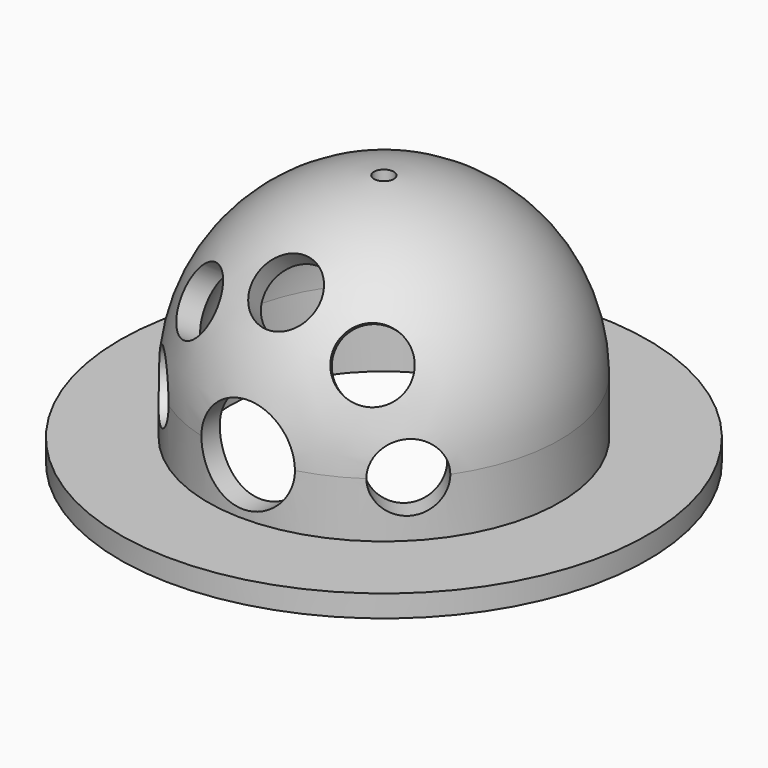
from build123d import *

# Parameters (mm, degrees)
F2_R             = 4.25
F3_DEPTH         = 50
F6_R             = 3
F7_DEPTH         = 25
F11_COPIES_COUNT = 3
F11_COPIES_ANGLE = 90
F13_R            = 3
F14_DEPTH        = 25
F16_R            = 0.9
F17_DEPTH        = 30.1


# Not quite as in the source:
# - a pattern or mirror of a feature is missing from the dataset's text; its kind, count and spacing are read off the source's solid


with BuildPart() as f1:
    # F0 (on Front) → F1 (revolve)
    with BuildSketch(Plane.XZ):
        with BuildLine():
            Line((-24, -7), (-14, -7))
            Line((-14, -7), (-14, 0))
            ThreePointArc((-14, 0), (-9.8994949366, 9.8994949366), (0, 14))
            Line((0, 14), (0, 16))
            ThreePointArc((0, 16), (-11.313708499, 11.313708499), (-16, 0))
            Line((-16, 0), (-16, -5))
            Line((-16, -5), (-24, -5))
            Line((-24, -5), (-24, -7))
        make_face()
    revolve(axis=Axis((0, 0, 15), (0, 0, -1)))

    # F2 (on Front) → F3 (cut)
    with BuildSketch(Plane.XZ):
        Circle(F2_R)
    extrude(amount=F3_DEPTH, mode=Mode.SUBTRACT)

    # F6 (on face) → F7 (cut)
    with BuildSketch(Plane(origin=(0, 0, 0), x_dir=(-0.7071067812, 0.7071067812, 0), z_dir=(0.7071067812, 0.7071067812, 0))):
        Circle(F6_R)
    extrude(amount=-F7_DEPTH, mode=Mode.SUBTRACT)

    # F10 (on face) → F11 (revolve, cut)
    with BuildSketch(Plane(origin=(0, 0, 0), x_dir=(0, -1, 0), z_dir=(-0.7071067812, 0, 0.7071067812))):
        Polygon((3.9985278842, 3.9985278842), (16.6846810101, 16.6846810101), (14.5633606666, 18.8060013537), (1.8772075407, 6.1198482278), align=None)
    f11 = revolve(axis=Axis((7.3126186329, -10.3416044472, 7.3126186329), (0.5, -0.7071067812, 0.5)), mode=Mode.SUBTRACT)

    # F11_copies: F11 ×3 about axis
    f11_copies_axis = Axis((0, 0, 0), (0, -1, 0))
    for i in range(1, F11_COPIES_COUNT):
        add(f11.rotate(f11_copies_axis, i * F11_COPIES_ANGLE / (F11_COPIES_COUNT - 1)), mode=Mode.SUBTRACT)

    # F13 (on face) → F14 (cut)
    with BuildSketch(Plane(origin=(0, 0, 0), x_dir=(0.7071067812, 0.7071067812, 0), z_dir=(0.7071067812, -0.7071067812, 0))):
        Circle(F13_R)
    extrude(amount=F14_DEPTH, mode=Mode.SUBTRACT)

    # F16 (on Top) → F17 (cut)
    with BuildSketch(Plane.XY):
        Circle(F16_R)
    extrude(amount=F17_DEPTH, mode=Mode.SUBTRACT)


solid = f1.part
